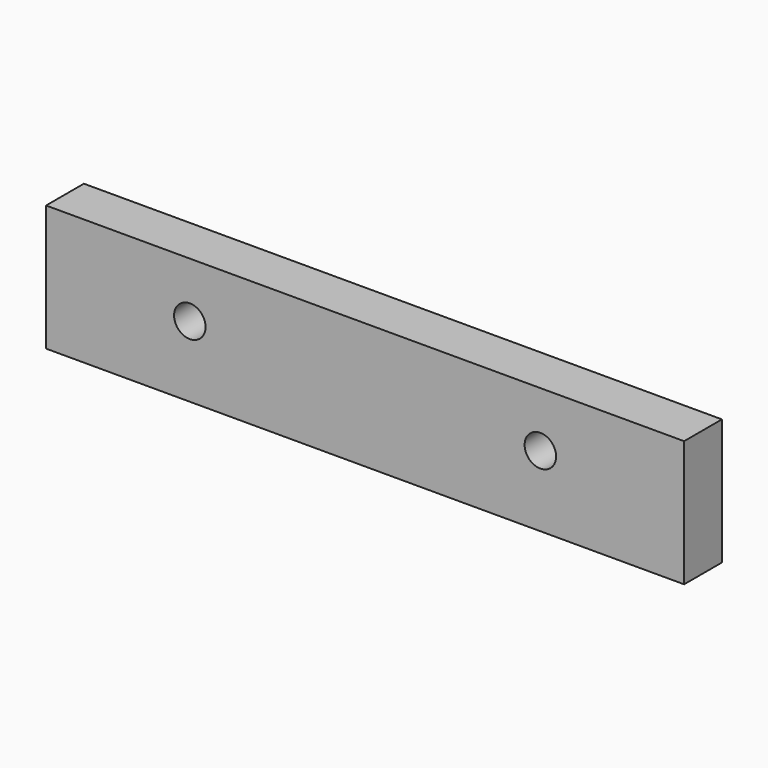
from build123d import *

# Parameters (mm, degrees)
F0_W     = 162
F0_H     = 32
F1_DEPTH = 12
F3_D     = 8


# Not quite as in the source:
# - a pattern or mirror of a feature is missing from the dataset's text; its kind, count and spacing are read off the source's solid


with BuildPart() as f1:
    # F0 (on Front) → F1 (new body)
    with BuildSketch(Plane.XZ):
        Rectangle(F0_W, F0_H)
    extrude(amount=-F1_DEPTH)

    # F3 (through all)
    with Locations(Plane.XZ):
        with Locations((-44.5, 2)):
            f3 = Hole(F3_D / 2)

    # F3_copies: F3 across plane
    add(f3.mirror(Plane(origin=(0, 0, 0), x_dir=(0, 0, 1), z_dir=(1, 0, 0))), mode=Mode.SUBTRACT)


solid = f1.part
